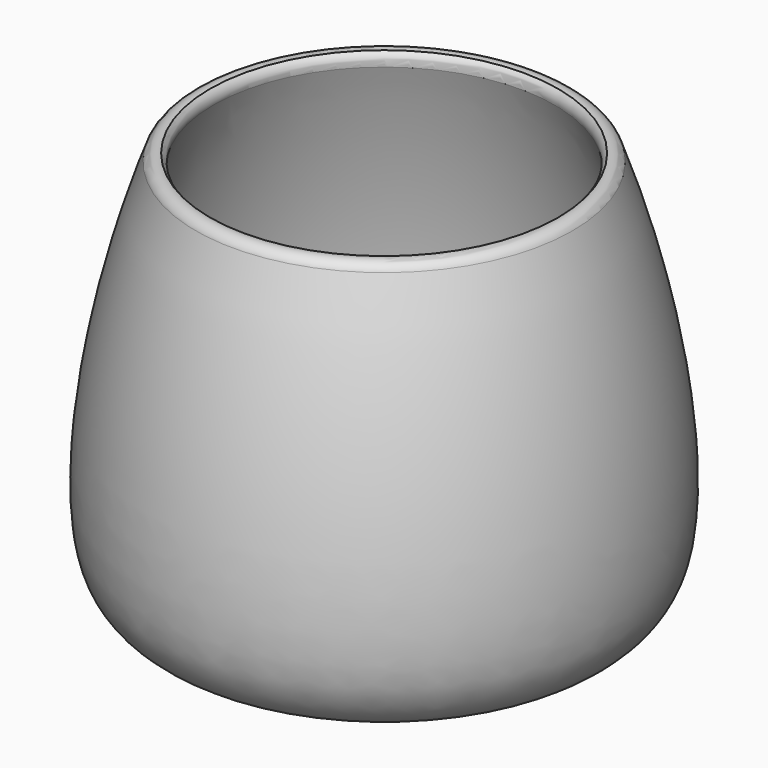
from build123d import *


# Not quite as in the source:
# - ends of sketch curves that miss each other by under 0.0002 mm in the source are joined
# - the dataset's text gives a spline's control points without its knots; the knots are read off the source's solid


with BuildPart() as f1:
    # F0 (on Front) → F1 (revolve)
    with BuildSketch(Plane.XZ):
        with BuildLine():
            Line((-50.0863976777, 0), (0, 0))
            Line((0, 0), (0, 4.8340512948))
            Line((0, 4.8340512948), (-48.5248765991, 4.8340512948))
            add(Edge.make_bspline(
                [(-48.5248765991, 4.8340512948), (-50.3395047187, 5.420222166), (-52.6065746829, 6.4311894859), (-54.8987261778, 7.9704561016), (-56.3195451599, 9.2221188831), (-57.5073659292, 10.5935290068), (-58.5149287339, 12.1253927354), (-59.3722749468, 13.8613674431), (-60.3307658744, 16.490607067), (-61.0160480255, 19.6278525262), (-61.3932597375, 22.8138450271), (-61.551529172, 24.7541931177), (-61.6743125207, 26.7756050679), (-61.7639687215, 29.4283073418), (-61.7693384185, 33.9139679968), (-61.5176985199, 39.9402724198), (-60.8079316474, 47.7324737119), (-59.3308579603, 58.7333237117), (-56.5175438769, 73.3821408075), (-51.9825972274, 90.54768366), (-48.3165372525, 101.5854259409), (-46.5234702366, 106.48663533)],
                knots=[0, 0, 0, 0, 0.0625, 0.09375, 0.125, 0.15625, 0.1875, 0.21875, 0.25, 0.3125, 0.34375, 0.359375, 0.375, 0.40625, 0.4375, 0.5, 0.5625, 0.625, 0.75, 0.875, 0.9777496991, 0.9777496991, 0.9777496991, 0.9777496991], degree=3))
            ThreePointArc((-46.5234702366, 106.48663533), (-46.4426852666, 108.4151215233), (-47.493727464, 110.0340356596))
            ThreePointArc((-47.493727464, 110.0340356596), (-49.8097373438, 109.8125516176), (-51.35292447, 108.0714225479))
            add(Edge.make_bspline(
                [(-50.0863976777, 0), (-62.653142504, 4.0593770604), (-71.3940131158, 26.9859179227), (-62.0996857499, 78.6374780387), (-51.35292447, 108.0714225479)],
                knots=[0, 0, 0, 0, 0.3716442727, 0.97664931, 0.97664931, 0.97664931, 0.97664931], degree=3))
        make_face()
    revolve(axis=Axis((0, 0, 2.4170256474), (0, 0, -1)))


solid = f1.part
